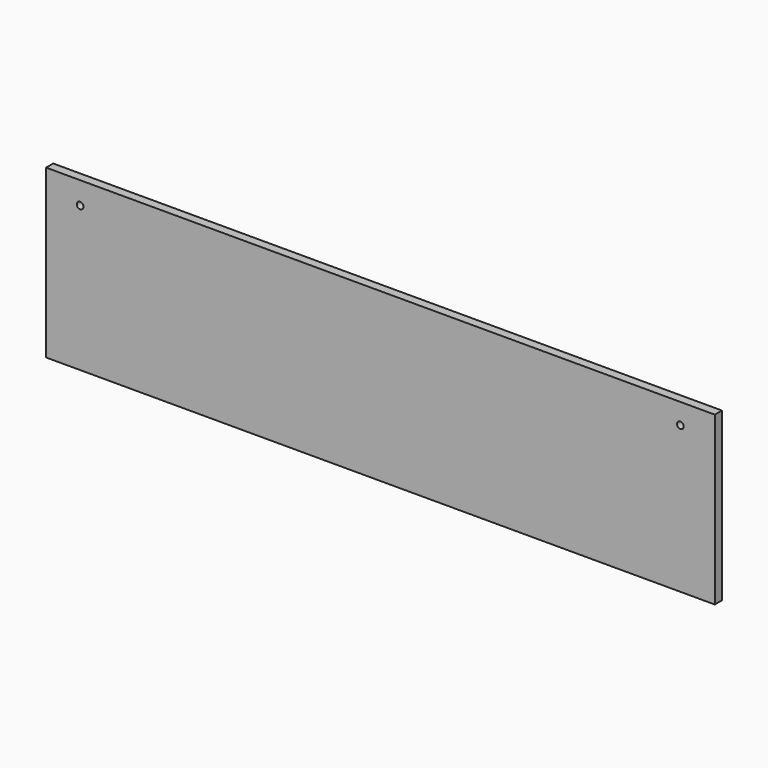
from build123d import *

# Parameters (mm, degrees)
F0_W         = 300
F0_H         = 75
F1_DEPTH     = 4
F2_TEXT_SIZE = 47.9358002647
F3_DEPTH     = 5
F5_D         = 3
F7_D         = 3


# Not quite as in the source:
# - Text() gives the source's letters only with a copy of the font that has no kerning and outlines rounded to 1/6400 em; it was checked with that copy


with BuildPart() as f1:
    # F0 (on Front) → F1 (new body)
    with BuildSketch(Plane.XZ):
        with Locations((150, 37.5)):
            Rectangle(F0_W, F0_H)
    extrude(amount=F1_DEPTH)

    # F2 (on face) → F3 (join)
    with BuildSketch(Plane(origin=(0, 0, 0), x_dir=(-1, 0, 0), z_dir=(0, 1, 0))):
        with Locations((-273.6833095551, 19.8116963729)):
            Text('Seriously?!', F2_TEXT_SIZE, font='Open Sans', font_style=FontStyle.BOLD, text_align=(TextAlign.LEFT, TextAlign.BOTTOM))
    extrude(amount=F3_DEPTH)

    # F5 (through all)
    with Locations(Plane(origin=(0, 0, 0), x_dir=(-1, 0, 0), z_dir=(0, 1, 0))):
        with Locations((-284.563601017, 65.7932087779)):
            Hole(F5_D / 2)

    # F7 (through all)
    with Locations(Plane(origin=(0, 0, 0), x_dir=(-1, 0, 0), z_dir=(0, 1, 0))):
        with Locations((-15.2631159872, 65)):
            Hole(F7_D / 2)


solid = f1.part
